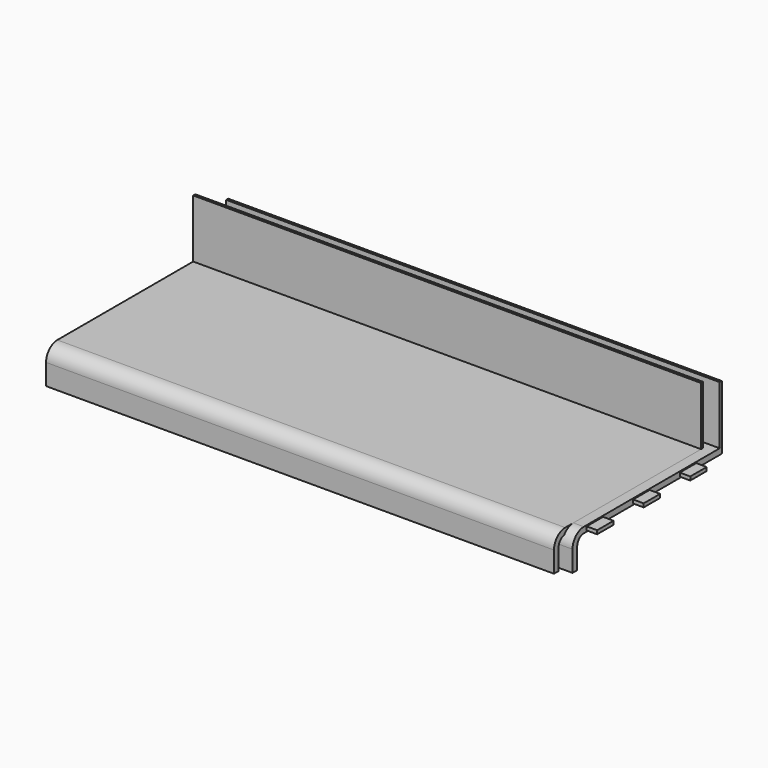
from build123d import *

# Parameters (mm, degrees)
F0_W        = 221.63532
F0_H        = 81.4832
F1_DEPTH    = 15.24
F2_T1_DEPTH = 480.2718812368
F3_R        = 6.1321024484
F4_T        = -2.54
F5_W        = 8.9602805674
F5_H        = 1.5747996354
F5_W_2      = 8.960280932
F5_H_2      = 1.5748
F6_DEPTH    = 4.572
F7_W        = 221.63532
F7_H        = 81.4832
F8_DEPTH    = 15.24
F9_R        = 6.1214
F10_T       = -2.54
F11_W       = 8.9602805674
F11_H       = 1.5609367454
F11_W_2     = 8.960280932
F11_H_2     = 1.56093711
F12_DEPTH   = 4.572
F13_W       = 215.3674113799
F13_H       = 1.1208840015
F14_DEPTH   = 25.4
F15_W       = 221.63532
F15_H       = 1.1208766
F16_DEPTH   = 25.4


# Not quite as in the source:
# - a fillet or chamfer that OpenCascade refuses, or shapes differently, is made with other operations: its cross-section is extruded or revolved along the edge and cut away or added


with BuildPart() as f1:
    # F0 (on Top) → F1 (new body)
    with BuildSketch(Plane.XY):
        with Locations((4.5526515504, 4.4273882142)):
            Rectangle(F0_W, F0_H)
    extrude(amount=F1_DEPTH)

    # F2: fillet of radius 93.8211674609 on 1 edges, made by hand

    # F2_s2 → F2_t1 (cut)
    with BuildSketch(Plane.XY.offset(-232.5159406184)):
        with BuildLine():
            ThreePointArc((-106.2650084496, 45.1689882142), (-75.0843912046, -13.0620671855), (-13.2586322022, -36.3142117858))
            Line((-13.2586322022, -36.3142117858), (-106.2650084496, -36.3142117858))
            Line((-106.2650084496, -36.3142117858), (-106.2650084496, 45.1689882142))
        make_face()
    extrude(amount=F2_T1_DEPTH, mode=Mode.SUBTRACT)

    # F3
    f3_edges = [f1.edges().sort_by_distance(p)[0] for p in [
        (51.05584, -36.314212, 15.24),
    ]]
    fillet(f3_edges, radius=F3_R)

    # F4
    f4_openings = [f1.faces().sort_by_distance(p)[0] for p in [
        (14.62211, 6.737734, 0),
        (4.817098, 45.168988, 7.604896),
        (115.370312, 4.684912, 7.579118),
    ]]
    offset(amount=F4_T, openings=f4_openings)

    # F5 (on face) → F6 (join)
    with BuildSketch(Plane.YZ.offset(115.3703115504)):
        with Locations((-24.1282563657, 13.97)):
            Rectangle(F5_W, F5_H)
        with Locations((1.2717436343, 13.97)):
            Rectangle(F5_W_2, F5_H_2)
        with Locations((26.6717436343, 13.97)):
            Rectangle(F5_W_2, F5_H_2)
    extrude(amount=F6_DEPTH)

    # F13 (on face) → F14 (join)
    with BuildSketch(Plane.XY.offset(15.24)):
        with Locations((7.6866024757, 44.5356499554)):
            Rectangle(F13_W, F13_H)
    extrude(amount=F14_DEPTH)


with BuildPart() as f8:
    # F7 (on Top) → F8 (new body)
    with BuildSketch(Plane.XY):
        Rectangle(F7_W, F7_H)
    extrude(amount=F8_DEPTH)

    # F9
    f9_edges = [f8.edges().sort_by_distance(p)[0] for p in [
        (0, -40.7416, 15.24),
    ]]
    fillet(f9_edges, radius=F9_R)

    # F10
    f10_openings = [f8.faces().sort_by_distance(p)[0] for p in [
        (0, 0, 0),
        (-110.81766, 0.256635, 7.579246),
        (110.81766, 0.256635, 7.579246),
        (0, 40.7416, 7.62),
    ]]
    offset(amount=F10_T, openings=f10_openings)

    # F11 (on face) → F12 (cut)
    with BuildSketch(Plane(origin=(-110.81766, 0, 0), x_dir=(0, -1, 0), z_dir=(-1, 0, 0))):
        with Locations((-22.3312906812, 13.9630684015)):
            Rectangle(F11_W, F11_H)
        with Locations((3.0687093188, 13.9630684015)):
            Rectangle(F11_W_2, F11_H_2)
        with Locations((28.4687093188, 13.9630684015)):
            Rectangle(F11_W_2, F11_H_2)
    extrude(amount=-F12_DEPTH, mode=Mode.SUBTRACT)

    # F15 (on face) → F16 (join)
    with BuildSketch(Plane.XY.offset(15.24)):
        with Locations((-3.3716e-06, 40.0574524351)):
            Rectangle(F15_W, F15_H)
    extrude(amount=F16_DEPTH)


solid = Compound([f1.part, f8.part])
